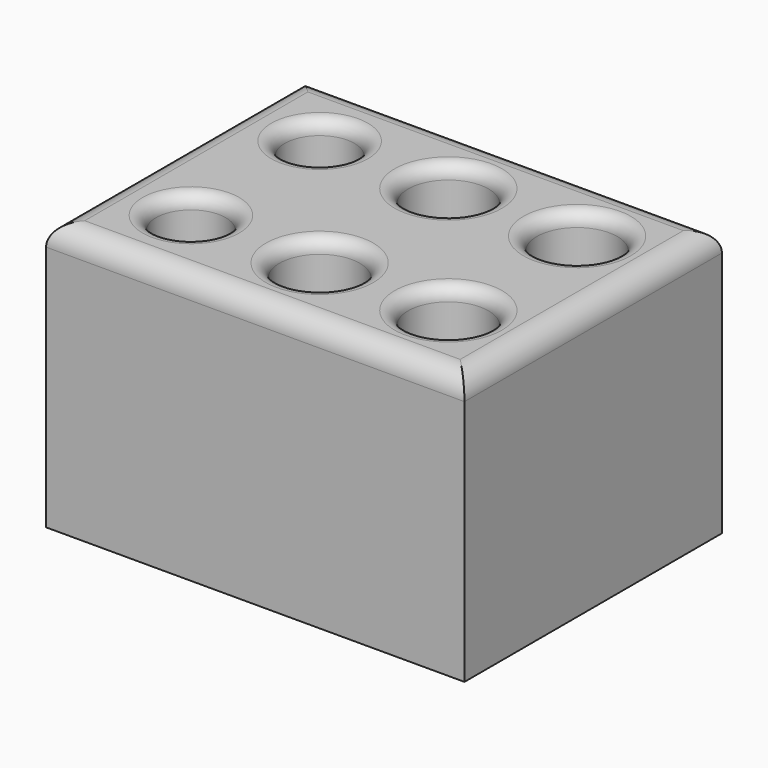
from build123d import *

# Parameters (mm, degrees)
F0_W     = 78
F0_H     = 60
F0_R     = 7.5
F0_R_2   = 6.5
F1_DEPTH = 50
F2_DEPTH = 47
F3_R     = 4
F4_R     = 2.5


# Not quite as in the source:
# - a feature names something its author has since deleted; it is built from what else it names


with BuildPart() as f1:
    # F0 (on Top) → F1 (new body)
    with BuildSketch(Plane.XY):
        Rectangle(F0_W, F0_H)
        with Locations((-24, -15)):
            Circle(F0_R, mode=Mode.SUBTRACT)
        with Locations((0, -15)):
            Circle(F0_R, mode=Mode.SUBTRACT)
        with Locations((24, -15)):
            Circle(F0_R, mode=Mode.SUBTRACT)
        with Locations((-24, 15)):
            Circle(F0_R, mode=Mode.SUBTRACT)
        with Locations((0, 15)):
            Circle(F0_R, mode=Mode.SUBTRACT)
        with Locations((24, 15)):
            Circle(F0_R, mode=Mode.SUBTRACT)
        with Locations((-24, 15)):
            Circle(F0_R)
        with Locations((-24, 15)):
            Circle(F0_R_2, mode=Mode.SUBTRACT)
        with Locations((-24, -15)):
            Circle(F0_R)
        with Locations((-24, -15)):
            Circle(F0_R_2, mode=Mode.SUBTRACT)
        with Locations((0, 15)):
            Circle(F0_R)
        with Locations((24, 15)):
            Circle(F0_R)
        with Locations((24, -15)):
            Circle(F0_R)
        with Locations((0, -15)):
            Circle(F0_R)
        with Locations((-24, 15)):
            Circle(F0_R_2)
        with Locations((-24, -15)):
            Circle(F0_R_2)
    extrude(amount=-F1_DEPTH)

    # F0 (on Top) → F2 (cut)
    with BuildSketch(Plane.XY):
        with Locations((-24, -15)):
            Circle(F0_R_2)
        with Locations((-24, 15)):
            Circle(F0_R_2)
        with Locations((0, 15)):
            Circle(F0_R)
        with Locations((24, -15)):
            Circle(F0_R)
        with Locations((24, 15)):
            Circle(F0_R)
        with Locations((0, -15)):
            Circle(F0_R)
    extrude(amount=-F2_DEPTH, mode=Mode.SUBTRACT)

    # F3
    f3_edges = [f1.edges().sort_by_distance(p)[0] for p in [
        (0, -30, 0),
        (39, 0, 0),
        (0, 30, 0),
        (-39, 0, 0),
    ]]
    fillet(f3_edges, radius=F3_R)

    # F4
    f4_edges = [f1.edges().sort_by_distance(p)[0] for p in [
        (16.5, -15, 0),
        (-7.5, 15, 0),
        (16.5, 15, 0),
        (-30.5, 15, 0),
        (-30.5, -15, 0),
        (16.5, -15, -47),
        (16.5, 15, -47),
        (-30.5, 15, -47),
        (-7.5, 15, -47),
        (-30.5, -15, -47),
        (-7.5, -15, 0),
    ]]
    fillet(f4_edges, radius=F4_R)


solid = f1.part
